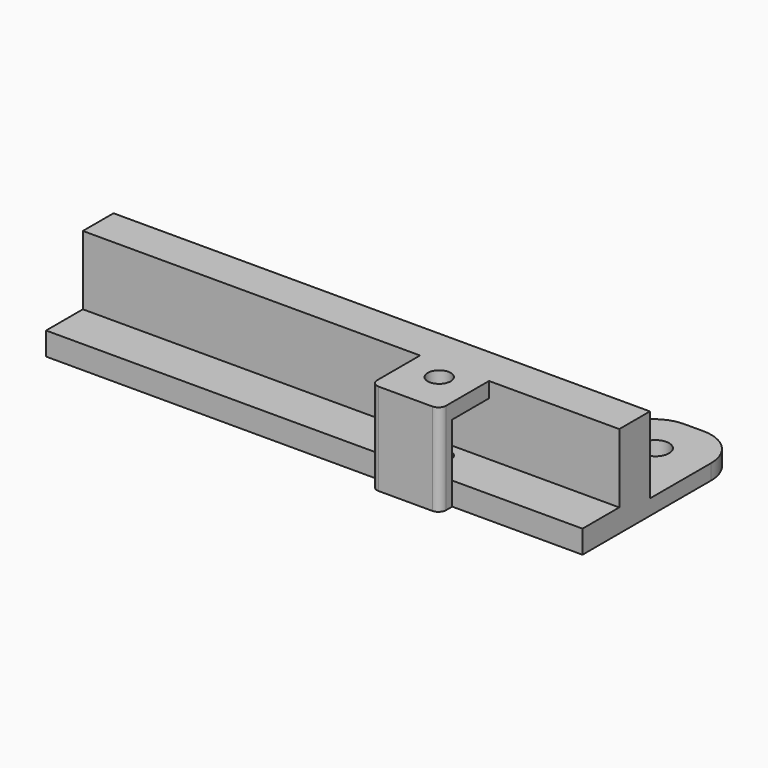
from build123d import *

# Parameters (mm, degrees)
F0_R      = 1.8
F1_DEPTH  = 2
F2_R      = 4.99999
F3_W      = 70
F3_H      = 5
F4_DEPTH  = 10
F5_W      = 70
F5_H      = 3
F6_DEPTH  = 6
F8_W      = 9
F8_H      = 2
F9_DEPTH  = 8
F10_W     = 9
F10_H     = 2
F11_DEPTH = 10
F7_R      = 1.5
F12_DEPTH = 12.001
F13_R     = 1


# Not quite as in the source:
# - a fillet or chamfer is up to 0.001 mm smaller than in the source, because OpenCascade refuses the exact size


with BuildPart() as f1:
    # F0 (on Top) → F1 (new body)
    with BuildSketch(Plane.XY):
        Polygon((-22.5, 10), (-35, 10), (-35, -10), (35, -10), (35, 10), (22.5, 10), (22.5, 0), (0, 0), (-22.5, 0), align=None)
        with Locations((-28.5, 4)):
            Circle(F0_R, mode=Mode.SUBTRACT)
        with Locations((28.5, 4)):
            Circle(F0_R, mode=Mode.SUBTRACT)
    extrude(amount=F1_DEPTH)

    # F2 (radius 5 in the source; OpenCascade refuses exactly that, so slightly less here)
    f2_edges = [f1.edges().sort_by_distance(p)[0] for p in [
        (22.5, 10, 1),
        (35, 10, 1),
        (-22.5, 10, 1),
        (-35, 10, 1),
        (-22.5, 0, 1),
        (22.5, 0, 1),
    ]]
    fillet(f2_edges, radius=F2_R)

    # F3 (on face) → F4 (join)
    with BuildSketch(Plane.XY.offset(2)):
        with Locations((0, -7.5)):
            Rectangle(F3_W, F3_H)
    extrude(amount=F4_DEPTH)

    # F5 (on face) → F6 (join)
    with BuildSketch(Plane.XZ.offset(10)):
        with Locations((0, 1.5)):
            Rectangle(F5_W, F5_H)
    extrude(amount=F6_DEPTH)

    # F8 (on face) → F9 (join)
    with BuildSketch(Plane.XZ.offset(10)):
        with Locations((13.5, 11)):
            Rectangle(F8_W, F8_H)
    extrude(amount=F9_DEPTH)

    # F10 (on face) → F11 (join)
    with BuildSketch(Plane(origin=(0, 0, 10), x_dir=(1, 0, 0), z_dir=(0, 0, -1))):
        with Locations((13.5, 17)):
            Rectangle(F10_W, F10_H)
    extrude(amount=F11_DEPTH)

    # F7 (on face) → F12 (cut, through all)
    with BuildSketch(Plane(origin=(0, 0, 0), x_dir=(1, 0, 0), z_dir=(0, 0, -1))):
        with Locations((13.5, 12.5)):
            Circle(F7_R)
    extrude(amount=-F12_DEPTH, mode=Mode.SUBTRACT)

    # F13
    f13_edges = [f1.edges().sort_by_distance(p)[0] for p in [
        (9, -18, 6),
        (18, -18, 6),
    ]]
    fillet(f13_edges, radius=F13_R)


solid = f1.part
